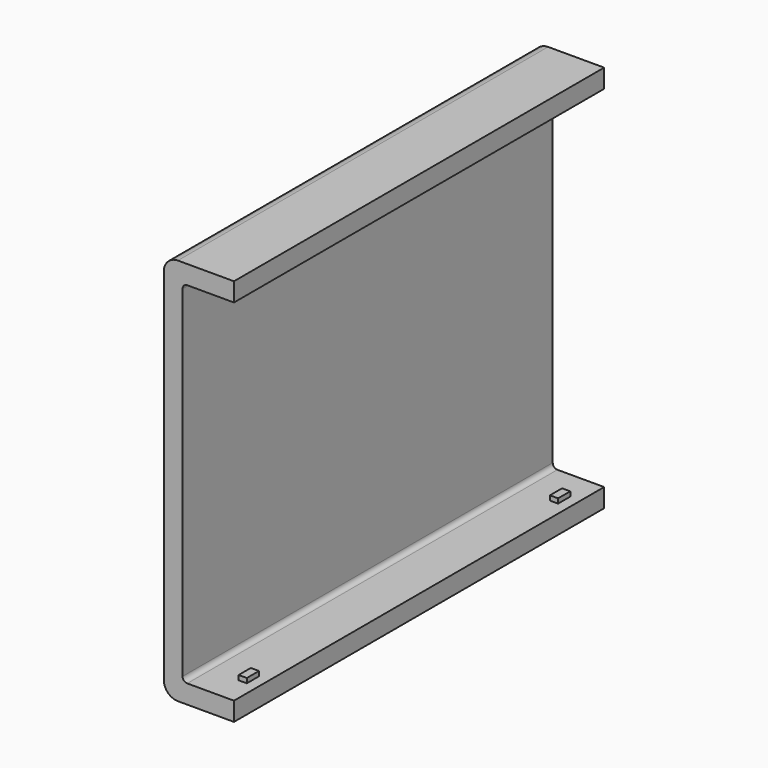
from build123d import *

# Parameters (mm, degrees)
F1_DEPTH      = 49.5
F1_DEPTH_BACK = 49.5
F2_W          = 1.75
F2_H          = 3.25
F3_DEPTH      = 1


# Not quite as in the source:
# - a pattern or mirror of a feature is missing from the dataset's text; its kind, count and spacing are read off the source's solid


with BuildPart() as f1:
    # F0 (on Front) → F1 (new body, two sides)
    with BuildSketch(Plane.XZ) as f1_sk:
        with BuildLine():
            ThreePointArc((3, 41.75), (0.8786796564, 40.8713203436), (0, 38.75))
            Line((0, 38.75), (0, -38.25))
            ThreePointArc((0, -38.25), (0.8786796564, -40.3713203436), (3, -41.25))
            Line((3, -41.25), (15, -41.25))
            Line((15, -41.25), (15, -37.25))
            Line((15, -37.25), (5, -37.25))
            ThreePointArc((5, -37.25), (4.2928932188, -36.9571067812), (4, -36.25))
            Line((4, -36.25), (4, 36.75))
            ThreePointArc((4, 36.75), (4.2928932188, 37.4571067812), (5, 37.75))
            Line((5, 37.75), (15, 37.75))
            Line((15, 37.75), (15, 41.75))
            Line((15, 41.75), (3, 41.75))
        make_face()
    extrude(amount=F1_DEPTH)
    extrude(f1_sk.sketch, amount=-F1_DEPTH_BACK)

    # F2 (on face) → F3 (join)
    with BuildSketch(Plane.XY.offset(-37.25)):
        with Locations((11.875, 41.625)):
            Rectangle(F2_W, F2_H)
        with Locations((11.875, -41.625)):
            Rectangle(F2_W, F2_H)
    f3 = extrude(amount=F3_DEPTH)

    # F3_copies: F3 across plane
    add(f3.mirror(Plane.XY))


solid = f1.part
